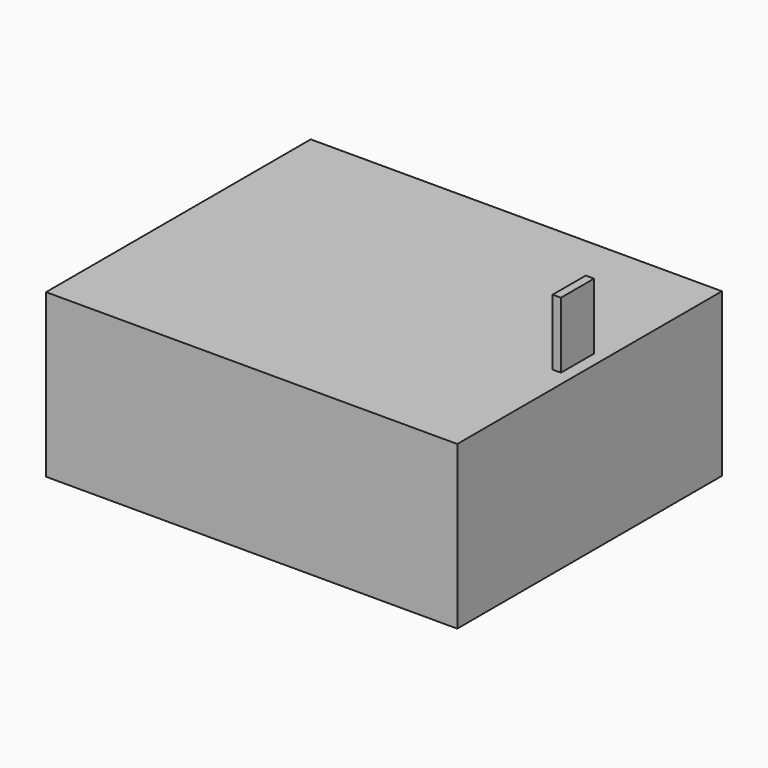
from build123d import *

# Parameters (mm, degrees)
F0_W     = 63.144043088
F0_H     = 24.9639227986
F1_DEPTH = 25.4
F2_W     = 1.27
F2_H     = 10.16
F3_DEPTH = 3.175
F4_W     = 10.16
F4_H     = 1.27
F5_DEPTH = 3.175


# Not quite as in the source:
# - a feature names something its author has since deleted; it is built from what else it names


with BuildPart() as f1:
    # F0 (on Front) → F1 (new body, symmetric)
    with BuildSketch(Plane.XZ):
        Rectangle(F0_W, F0_H)
    extrude(amount=F1_DEPTH, both=True)

    # F2 (on Front) → F3 (join, symmetric)
    with BuildSketch(Plane.XZ):
        with Locations((29.0800049829, 17.5400783525)):
            Rectangle(F2_W, F2_H)
    extrude(amount=F3_DEPTH, both=True)

    # F4 (on Front) → F5 (join, symmetric)
    with BuildSketch(Plane.XZ):
        with Locations((-36.6476550698, -9.8343824477)):
            Rectangle(F4_W, F4_H)
    extrude(amount=F5_DEPTH, both=True)


solid = f1.part
